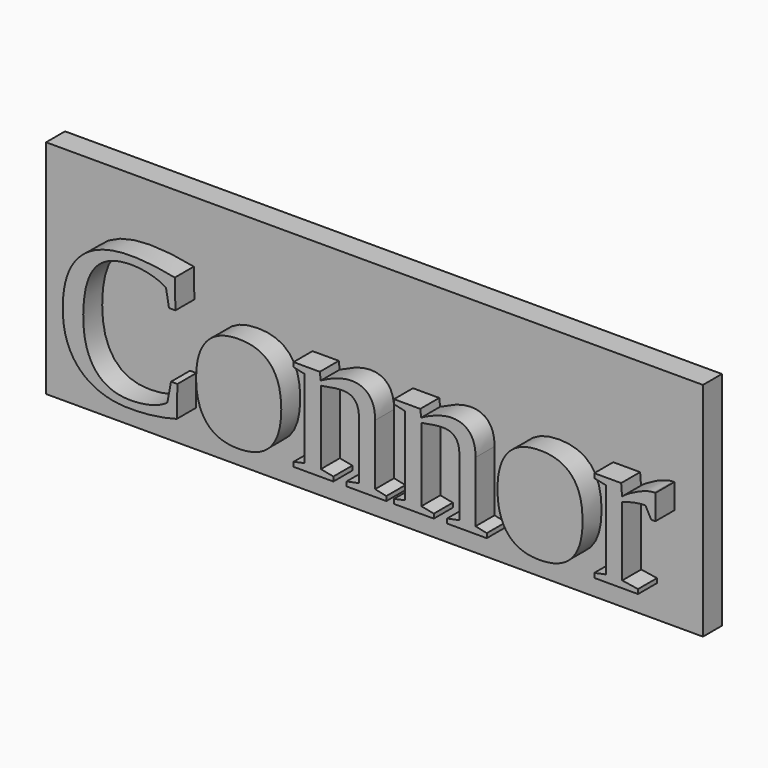
from build123d import *

# Parameters (mm, degrees)
F0_TEXT_SIZE = 107.5855352812
F1_DEPTH     = 25.4
F2_W         = 351.7773300409
F2_H         = 118.6904832721
F3_DEPTH     = 12.7


# Not quite as in the source:
# - Text() gives the source's letters only with a copy of the font that has no kerning and outlines rounded to 1/6400 em; it was checked with that copy


with BuildPart() as f1:
    # F0 (on Front) → F1 (new body)
    with BuildSketch(Plane.XZ):
        with BuildLine():
            add(Edge.make_bspline(
                [(-76.3625056295, -24.0002133214), (-73.000457652, -18.8478747958), (-73.000457652, -7.299239993)],
                knots=[0, 0, 0, 1, 1, 1], degree=2))
            add(Edge.make_bspline(
                [(-73.000457652, -7.299239993), (-73.000457652, 4.0476719312), (-76.3120749099, 9.1495797371)],
                knots=[0, 0, 0, 1, 1, 1], degree=2))
            add(Edge.make_bspline(
                [(-76.3120749099, 9.1495797371), (-79.6236921677, 14.251487543), (-86.6671826807, 14.251487543)],
                knots=[0, 0, 0, 1, 1, 1], degree=2))
            add(Edge.make_bspline(
                [(-86.6671826807, 14.251487543), (-93.5425707948, 14.251487543), (-96.6188446942, 9.3597077357)],
                knots=[0, 0, 0, 1, 1, 1], degree=2))
            add(Edge.make_bspline(
                [(-96.6188446942, 9.3597077357), (-99.6951185936, 4.4679279284), (-99.6951185936, -7.299239993)],
                knots=[0, 0, 0, 1, 1, 1], degree=2))
            add(Edge.make_bspline(
                [(-99.6951185936, -7.299239993), (-99.6951185936, -19.2177000734), (-96.5684139745, -24.1851259602)],
                knots=[0, 0, 0, 1, 1, 1], degree=2))
            add(Edge.make_bspline(
                [(-96.5684139745, -24.1851259602), (-93.4417093554, -29.152551847), (-86.6671826807, -29.152551847)],
                knots=[0, 0, 0, 1, 1, 1], degree=2))
            add(Edge.make_bspline(
                [(-86.6671826807, -29.152551847), (-79.7245536071, -29.152551847), (-76.3625056295, -24.0002133214)],
                knots=[0, 0, 0, 1, 1, 1], degree=2))
        make_face()
        with BuildLine():
            add(Edge.make_bspline(
                [(85.0157972923, -24.0002133214), (88.3778452699, -18.8478747958), (88.3778452699, -7.299239993)],
                knots=[0, 0, 0, 1, 1, 1], degree=2))
            add(Edge.make_bspline(
                [(88.3778452699, -7.299239993), (88.3778452699, 4.0476719312), (85.066228012, 9.1495797371)],
                knots=[0, 0, 0, 1, 1, 1], degree=2))
            add(Edge.make_bspline(
                [(85.066228012, 9.1495797371), (81.7546107541, 14.251487543), (74.7111202412, 14.251487543)],
                knots=[0, 0, 0, 1, 1, 1], degree=2))
            add(Edge.make_bspline(
                [(74.7111202412, 14.251487543), (67.8357321271, 14.251487543), (64.7594582277, 9.3597077357)],
                knots=[0, 0, 0, 1, 1, 1], degree=2))
            add(Edge.make_bspline(
                [(64.7594582277, 9.3597077357), (61.6831843282, 4.4679279284), (61.6831843282, -7.299239993)],
                knots=[0, 0, 0, 1, 1, 1], degree=2))
            add(Edge.make_bspline(
                [(61.6831843282, -7.299239993), (61.6831843282, -19.2177000734), (64.8098889473, -24.1851259602)],
                knots=[0, 0, 0, 1, 1, 1], degree=2))
            add(Edge.make_bspline(
                [(64.8098889473, -24.1851259602), (67.9365935664, -29.152551847), (74.7111202412, -29.152551847)],
                knots=[0, 0, 0, 1, 1, 1], degree=2))
            add(Edge.make_bspline(
                [(74.7111202412, -29.152551847), (81.6537493148, -29.152551847), (85.0157972923, -24.0002133214)],
                knots=[0, 0, 0, 1, 1, 1], degree=2))
        make_face()
        with Locations((-185.0070860237, -32.2456359863)):
            Text('Connor', F0_TEXT_SIZE, font='Tinos', text_align=(TextAlign.LEFT, TextAlign.BOTTOM))
    extrude(amount=F1_DEPTH)


with BuildPart() as f3:
    # F2 (on Front) → F3 (new body)
    with BuildSketch(Plane.XZ):
        with Locations((-23.7731412053, 9.8531879485)):
            Rectangle(F2_W, F2_H)
    extrude(amount=F3_DEPTH)


solid = Compound([f1.part, f3.part])
